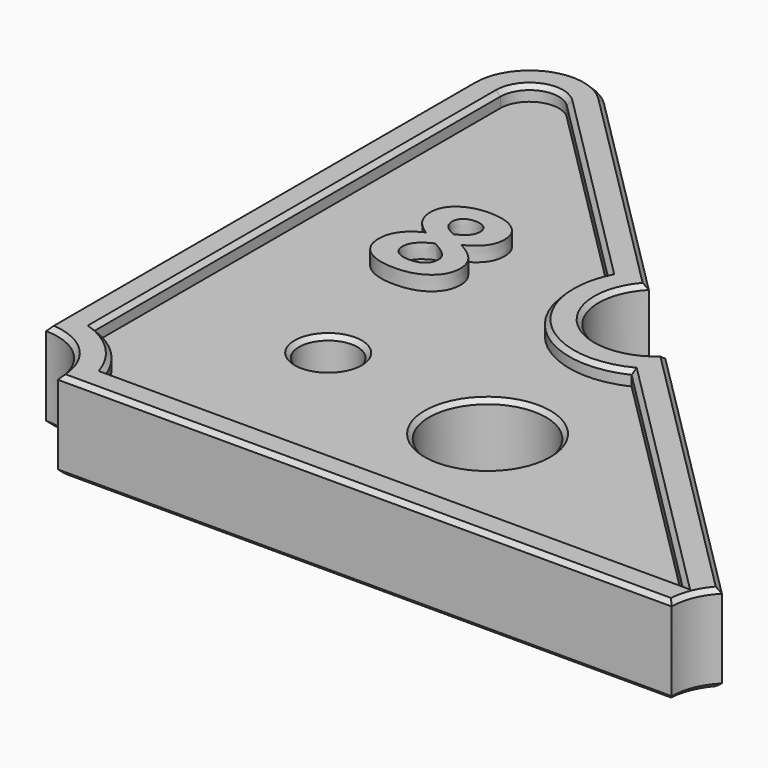
from build123d import *

# Parameters (mm, degrees)
F0_R         = 2
F0_R_2       = 4
F0_TEXT_SIZE = 11.1111111111
F1_DEPTH     = 5
F3_DEPTH     = 1
F4_SIZE      = 0.3


# Not quite as in the source:
# - Text() gives the source's letters only with a copy of the font that has no kerning and outlines rounded to 1/6400 em; it was checked with that copy


with BuildPart() as f1:
    # F0 (on Top) → F1 (new body)
    with BuildSketch(Plane.XY):
        with BuildLine():
            ThreePointArc((-18.1715728753, 18.1715728753), (-22.5307337295, 19.0386638806), (-25, 15.3431457505))
            Line((-25, 15.3431457505), (-25, -21))
            ThreePointArc((-25, -21), (-22.1715728753, -22.1715728753), (-21, -25))
            Line((-21, -25), (21, -25))
            ThreePointArc((21, -25), (21.30448187, -23.4692662705), (22.1715728753, -22.1715728753))
            Line((22.1715728753, -22.1715728753), (2.8284271247, -2.8284271247))
            ThreePointArc((2.8284271247, -2.8284271247), (-2.8284271247, -2.8284271247), (-2.8284271247, 2.8284271247))
            Line((-2.8284271247, 2.8284271247), (-18.1715728753, 18.1715728753))
        make_face()
        with Locations((-12.5, -12.5)):
            Circle(F0_R, mode=Mode.SUBTRACT)
        with Locations((0, -14.5)):
            Circle(F0_R_2, mode=Mode.SUBTRACT)
        with BuildLine():
            add(Edge.make_bspline(
                [(-16.4982638889, 3.5086805556), (-15.7934027778, 4.0347222222), (-14.6597222222, 4.0347222222)],
                knots=[0, 0, 0, 1, 1, 1], degree=2))
            add(Edge.make_bspline(
                [(-14.6597222222, 4.0347222222), (-13.5190972222, 4.0347222222), (-12.8220486111, 3.5164930556)],
                knots=[0, 0, 0, 1, 1, 1], degree=2))
            add(Edge.make_bspline(
                [(-12.8220486111, 3.5164930556), (-12.125, 2.9982638889), (-12.125, 2.1197916667)],
                knots=[0, 0, 0, 1, 1, 1], degree=2))
            add(Edge.make_bspline(
                [(-12.125, 2.1197916667), (-12.125, 1.5121527778), (-12.4618055556, 1.0373263889)],
                knots=[0, 0, 0, 1, 1, 1], degree=2))
            add(Edge.make_bspline(
                [(-12.4618055556, 1.0373263889), (-12.7986111111, 0.5625), (-13.546875, 0.1892361111)],
                knots=[0, 0, 0, 1, 1, 1], degree=2))
            add(Edge.make_bspline(
                [(-13.546875, 0.1892361111), (-12.6579861111, -0.2881944444), (-12.2699652778, -0.8064236111)],
                knots=[0, 0, 0, 1, 1, 1], degree=2))
            add(Edge.make_bspline(
                [(-12.2699652778, -0.8064236111), (-11.8819444444, -1.3246527778), (-11.8819444444, -1.9444444444)],
                knots=[0, 0, 0, 1, 1, 1], degree=2))
            add(Edge.make_bspline(
                [(-11.8819444444, -1.9444444444), (-11.8819444444, -2.9201388889), (-12.6467013889, -3.5147569444)],
                knots=[0, 0, 0, 1, 1, 1], degree=2))
            add(Edge.make_bspline(
                [(-12.6467013889, -3.5147569444), (-13.4114583333, -4.109375), (-14.6597222222, -4.109375)],
                knots=[0, 0, 0, 1, 1, 1], degree=2))
            add(Edge.make_bspline(
                [(-14.6597222222, -4.109375), (-15.9618055556, -4.109375), (-16.7048611111, -3.5555555556)],
                knots=[0, 0, 0, 1, 1, 1], degree=2))
            add(Edge.make_bspline(
                [(-16.7048611111, -3.5555555556), (-17.4479166667, -3.0017361111), (-17.4479166667, -1.9878472222)],
                knots=[0, 0, 0, 1, 1, 1], degree=2))
            add(Edge.make_bspline(
                [(-17.4479166667, -1.9878472222), (-17.4479166667, -1.3090277778), (-17.0868055556, -0.7829861111)],
                knots=[0, 0, 0, 1, 1, 1], degree=2))
            add(Edge.make_bspline(
                [(-17.0868055556, -0.7829861111), (-16.7256944444, -0.2569444444), (-15.9288194444, 0.1458333333)],
                knots=[0, 0, 0, 1, 1, 1], degree=2))
            add(Edge.make_bspline(
                [(-15.9288194444, 0.1458333333), (-16.6076388889, 0.5729166667), (-16.9053819444, 1.0616319444)],
                knots=[0, 0, 0, 1, 1, 1], degree=2))
            add(Edge.make_bspline(
                [(-16.9053819444, 1.0616319444), (-17.203125, 1.5503472222), (-17.203125, 2.1302083333)],
                knots=[0, 0, 0, 1, 1, 1], degree=2))
            add(Edge.make_bspline(
                [(-17.203125, 2.1302083333), (-17.203125, 2.9826388889), (-16.4982638889, 3.5086805556)],
                knots=[0, 0, 0, 1, 1, 1], degree=2))
        make_face(mode=Mode.SUBTRACT)
        with Locations((-17.8385416667, -4)):
            Text('8', F0_TEXT_SIZE, font='Open Sans', font_style=FontStyle.BOLD, text_align=(TextAlign.LEFT, TextAlign.BOTTOM))
        with BuildLine():
            add(Edge.make_bspline(
                [(-13.9756944444, 2.5920138889), (-14.2465277778, 2.8090277778), (-14.6701388889, 2.8090277778)],
                knots=[0, 0, 0, 1, 1, 1], degree=2))
            add(Edge.make_bspline(
                [(-14.6701388889, 2.8090277778), (-15.0989583333, 2.8090277778), (-15.3619791667, 2.5894097222)],
                knots=[0, 0, 0, 1, 1, 1], degree=2))
            add(Edge.make_bspline(
                [(-15.3619791667, 2.5894097222), (-15.625, 2.3697916667), (-15.625, 2)],
                knots=[0, 0, 0, 1, 1, 1], degree=2))
            add(Edge.make_bspline(
                [(-15.625, 2), (-15.625, 1.6753472222), (-15.4157986111, 1.4175347222)],
                knots=[0, 0, 0, 1, 1, 1], degree=2))
            add(Edge.make_bspline(
                [(-15.4157986111, 1.4175347222), (-15.2065972222, 1.1597222222), (-14.6597222222, 0.8888888889)],
                knots=[0, 0, 0, 1, 1, 1], degree=2))
            add(Edge.make_bspline(
                [(-14.6597222222, 0.8888888889), (-14.1267361111, 1.1371527778), (-13.9157986111, 1.3975694444)],
                knots=[0, 0, 0, 1, 1, 1], degree=2))
            add(Edge.make_bspline(
                [(-13.9157986111, 1.3975694444), (-13.7048611111, 1.6579861111), (-13.7048611111, 2)],
                knots=[0, 0, 0, 1, 1, 1], degree=2))
            add(Edge.make_bspline(
                [(-13.7048611111, 2), (-13.7048611111, 2.375), (-13.9756944444, 2.5920138889)],
                knots=[0, 0, 0, 1, 1, 1], degree=2))
        make_face()
        with BuildLine():
            add(Edge.make_bspline(
                [(-14.7413194444, -0.5434027778), (-15.8958333333, -1.0763888889), (-15.8958333333, -1.8888888889)],
                knots=[0, 0, 0, 1, 1, 1], degree=2))
            add(Edge.make_bspline(
                [(-15.8958333333, -1.8888888889), (-15.8958333333, -2.3559027778), (-15.5703125, -2.6163194444)],
                knots=[0, 0, 0, 1, 1, 1], degree=2))
            add(Edge.make_bspline(
                [(-15.5703125, -2.6163194444), (-15.2447916667, -2.8767361111), (-14.6805555556, -2.8767361111)],
                knots=[0, 0, 0, 1, 1, 1], degree=2))
            add(Edge.make_bspline(
                [(-14.6805555556, -2.8767361111), (-14.0572916667, -2.8767361111), (-13.7482638889, -2.6085069444)],
                knots=[0, 0, 0, 1, 1, 1], degree=2))
            add(Edge.make_bspline(
                [(-13.7482638889, -2.6085069444), (-13.4392361111, -2.3402777778), (-13.4392361111, -1.9010416667)],
                knots=[0, 0, 0, 1, 1, 1], degree=2))
            add(Edge.make_bspline(
                [(-13.4392361111, -1.9010416667), (-13.4392361111, -1.5364583333), (-13.7456597222, -1.2196180556)],
                knots=[0, 0, 0, 1, 1, 1], degree=2))
            add(Edge.make_bspline(
                [(-13.7456597222, -1.2196180556), (-14.0520833333, -0.9027777778), (-14.7413194444, -0.5434027778)],
                knots=[0, 0, 0, 1, 1, 1], degree=2))
        make_face()
    extrude(amount=-F1_DEPTH)

    # F0 (on Top) + F2 (on face) → F3 (join)
    with BuildSketch(Plane.XY):
        with Locations((-17.8385416667, -4)):
            Text('8', F0_TEXT_SIZE, font='Open Sans', font_style=FontStyle.BOLD, text_align=(TextAlign.LEFT, TextAlign.BOTTOM))
    with BuildSketch(Plane.XY):
        with BuildLine():
            ThreePointArc((21, -25), (21.30448187, -23.4692662705), (22.1715728753, -22.1715728753))
            Line((22.1715728753, -22.1715728753), (2.8284271247, -2.8284271247))
            ThreePointArc((2.8284271247, -2.8284271247), (-2.8284271247, -2.8284271247), (-2.8284271247, 2.8284271247))
            Line((-2.8284271247, 2.8284271247), (-18.1715728753, 18.1715728753))
            ThreePointArc((-18.1715728753, 18.1715728753), (-22.5307337295, 19.0386638806), (-25, 15.3431457505))
            Line((-25, 15.3431457505), (-25, -21))
            ThreePointArc((-25, -21), (-22.1715728753, -22.1715728753), (-21, -25))
            Line((-21, -25), (21, -25))
        make_face()
        with BuildLine():
            Line((2.5857864376, -5.4142135624), (20.1715728753, -23))
            Line((20.1715728753, -23), (-19.3431457505, -23))
            ThreePointArc((-19.3431457505, -23), (-20.7573593129, -20.7573593129), (-23, -19.3431457505))
            Line((-23, -19.3431457505), (-23, 15.3431457505))
            ThreePointArc((-23, 15.3431457505), (-21.7653668647, 17.1909048155), (-19.5857864376, 16.7573593129))
            Line((-19.5857864376, 16.7573593129), (-5.4142135624, 2.5857864376))
            ThreePointArc((-5.4142135624, 2.5857864376), (-4.2426406871, -4.2426406871), (2.5857864376, -5.4142135624))
        make_face(mode=Mode.SUBTRACT)
    extrude(amount=F3_DEPTH)

    # F4
    f4_edges = [f1.edges().sort_by_distance(p)[0] for p in [
        (-22.171573, -22.171573, 1),
        (0, -25, 1),
        (21.304482, -23.469266, 1),
        (12.5, -12.5, 1),
        (-2.828427, -2.828427, 1),
        (-10.5, 10.5, 1),
        (-22.530734, 19.038664, 1),
        (-25, -2.828427, 1),
        (-12.5, 9.671573, 1),
        (-4.242641, -4.242641, 1),
        (11.37868, -14.207107, 1),
        (0.414214, -23, 1),
        (-20.757359, -20.757359, 1),
        (-23, -2, 1),
        (-21.765367, 17.190905, 1),
        (-14.5, -12.5, 0),
        (-4, -14.5, 0),
        (12.5, -12.5, -5),
        (-2.828427, -2.828427, -5),
        (-10.5, 10.5, -5),
        (-22.530734, 19.038664, -5),
        (-25, -2.828427, -5),
        (-22.171573, -22.171573, -5),
        (0, -25, -5),
        (21.304482, -23.469266, -5),
        (-14.5, -12.5, -5),
        (-4, -14.5, -5),
    ]]
    chamfer(f4_edges, length=F4_SIZE)


solid = f1.part
